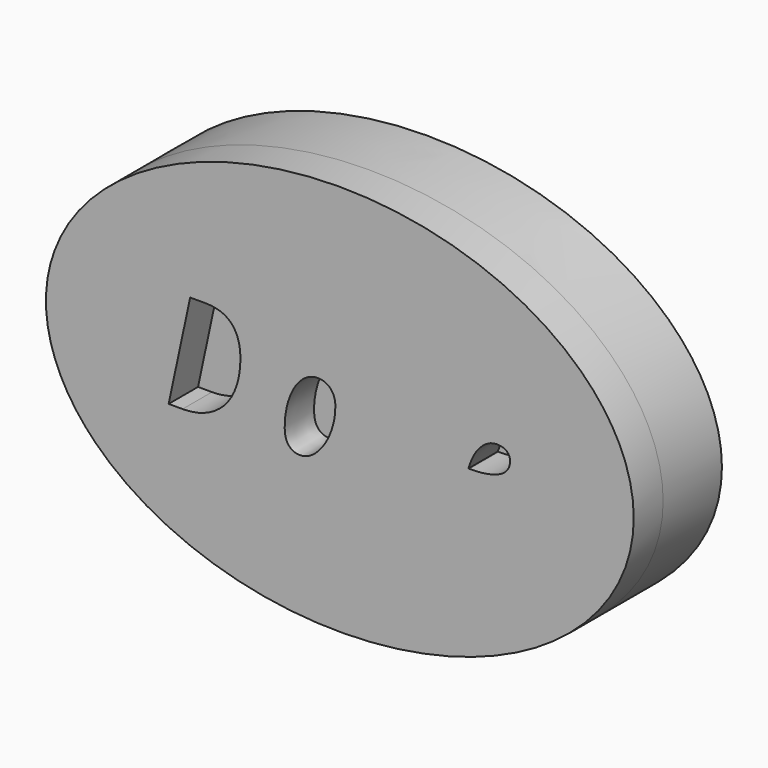
from build123d import *

# Parameters (mm, degrees)
F1_DEPTH     = 9.525
F2_TEXT_SIZE = 22.8748328995
F3_DEPTH     = 4.7625


# Not quite as in the source:
# - Text() gives the source's letters only with a copy of the font that has no kerning and outlines rounded to 1/6400 em; it was checked with that copy


with BuildPart() as f1:
    # F0 (on Front) → F1 (new body)
    with BuildSketch(Plane.XZ):
        with BuildLine():
            add(Edge.make_bspline(
                [(38.1, 0), (38.1, 43.9940905122), (-19.05, 21.9970452561), (-76.2, 0), (-19.05, -21.9970452561), (38.1, -43.9940905122), (38.1, 0)],
                knots=[0, 0, 0, 2.0943951024, 2.0943951024, 4.1887902048, 4.1887902048, 6.2831853072, 6.2831853072, 6.2831853072], degree=2, weights=[1, 0.5, 1, 0.5, 1, 0.5, 1]))
        make_face()
    extrude(amount=-F1_DEPTH)

    # F2 (on face) → F3 (join)
    with BuildSketch(Plane.XZ):
        with BuildLine():
            add(Edge.make_bspline(
                [(38.1, 0), (38.1, 43.9940905122), (-19.05, 21.9970452561), (-76.2, 0), (-19.05, -21.9970452561), (38.1, -43.9940905122), (38.1, 0)],
                knots=[0, 0, 0, 2.0943951024, 2.0943951024, 4.1887902048, 4.1887902048, 6.2831853072, 6.2831853072, 6.2831853072], degree=2, weights=[1, 0.5, 1, 0.5, 1, 0.5, 1]))
        make_face()
        with BuildLine():
            add(Edge.make_bspline(
                [(-12.4810807008, 6.4246112714), (-10.8780553015, 4.7536762119), (-10.8780553015, 1.5619221839)],
                knots=[0, 0, 0, 1, 1, 1], degree=2))
            add(Edge.make_bspline(
                [(-10.8780553015, 1.5619221839), (-10.8780553015, -1.3546190108), (-12.0521775839, -3.5884894111)],
                knots=[0, 0, 0, 1, 1, 1], degree=2))
            add(Edge.make_bspline(
                [(-12.0521775839, -3.5884894111), (-13.2262998663, -5.8223598114), (-15.4029831844, -7.0286498276)],
                knots=[0, 0, 0, 1, 1, 1], degree=2))
            add(Edge.make_bspline(
                [(-15.4029831844, -7.0286498276), (-17.5796665025, -8.2349398438), (-20.5069302751, -8.2349398438)],
                knots=[0, 0, 0, 1, 1, 1], degree=2))
            Line((-20.5069302751, -8.2349398438), (-24.4385421797, -8.2349398438))
            Line((-24.4385421797, -8.2349398438), (-20.9894462816, 8.0955463308))
            Line((-20.9894462816, 8.0955463308), (-17.1686343488, 8.0955463308))
            add(Edge.make_bspline(
                [(-17.1686343488, 8.0955463308), (-14.0841061, 8.0955463308), (-12.4810807008, 6.4246112714)],
                knots=[0, 0, 0, 1, 1, 1], degree=2))
        make_face(mode=Mode.SUBTRACT)
        with BuildLine():
            add(Edge.make_bspline(
                [(-6.0868500668, 3.102399212), (-4.6911278407, 4.2318440864), (-3.0255540702, 4.2318440864)],
                knots=[0, 0, 0, 1, 1, 1], degree=2))
            add(Edge.make_bspline(
                [(-3.0255540702, 4.2318440864), (-1.9997607824, 4.2318440864), (-1.1955674383, 3.6778442271)],
                knots=[0, 0, 0, 1, 1, 1], degree=2))
            add(Edge.make_bspline(
                [(-1.1955674383, 3.6778442271), (-0.3913740941, 3.1238443678), (0.0553999859, 2.0873285021)],
                knots=[0, 0, 0, 1, 1, 1], degree=2))
            Line((0.0553999859, 2.0873285021), (0.1804967283, 2.0873285021))
            Line((0.1804967283, 2.0873285021), (0.9275029902, 4.00666995))
            Line((0.9275029902, 4.00666995), (2.3464574685, 4.00666995))
            Line((2.3464574685, 4.00666995), (-0.2555547738, -8.2349398438))
            Line((-0.2555547738, -8.2349398438), (-1.7424189123, -8.2349398438))
            Line((-1.7424189123, -8.2349398438), (-1.4493351157, -5.9009920495))
            Line((-1.4493351157, -5.9009920495), (-1.5386899318, -5.9009920495))
            add(Edge.make_bspline(
                [(-1.5386899318, -5.9009920495), (-3.5402378105, -8.4601139802), (-5.7526630549, -8.4601139802)],
                knots=[0, 0, 0, 1, 1, 1], degree=2))
            add(Edge.make_bspline(
                [(-5.7526630549, -8.4601139802), (-7.3038626609, -8.4601139802), (-8.1866882432, -7.3539013579)],
                knots=[0, 0, 0, 1, 1, 1], degree=2))
            add(Edge.make_bspline(
                [(-8.1866882432, -7.3539013579), (-9.0695138254, -6.2476887357), (-9.0695138254, -4.3247730951)],
                knots=[0, 0, 0, 1, 1, 1], degree=2))
            add(Edge.make_bspline(
                [(-9.0695138254, -4.3247730951), (-9.0695138254, -2.0015478787), (-8.2760430592, -0.0142967706)],
                knots=[0, 0, 0, 1, 1, 1], degree=2))
            add(Edge.make_bspline(
                [(-8.2760430592, -0.0142967706), (-7.482572293, 1.9729543376), (-6.0868500668, 3.102399212)],
                knots=[0, 0, 0, 1, 1, 1], degree=2))
        make_face(mode=Mode.SUBTRACT)
        with BuildLine():
            Line((7.7971012453, -8.2349398438), (5.2522760853, -8.2349398438))
            Line((5.2522760853, -8.2349398438), (3.8547667628, 4.00666995))
            Line((3.8547667628, 4.00666995), (5.7312178991, 4.00666995))
            Line((5.7312178991, 4.00666995), (6.4460564272, -2.8414831492))
            add(Edge.make_bspline(
                [(6.4460564272, -2.8414831492), (6.7141208753, -5.7222824175), (6.7141208753, -6.8838950257)],
                knots=[0, 0, 0, 1, 1, 1], degree=2))
            Line((6.7141208753, -6.8838950257), (6.7820305354, -6.8838950257))
            add(Edge.make_bspline(
                [(6.7820305354, -6.8838950257), (8.2009850137, -3.8100893548), (8.7800042215, -2.7378315627)],
                knots=[0, 0, 0, 1, 1, 1], degree=2))
            Line((8.7800042215, -2.7378315627), (12.4113839443, 4.00666995))
            Line((12.4113839443, 4.00666995), (14.3986350524, 4.00666995))
            Line((14.3986350524, 4.00666995), (7.7971012453, -8.2349398438))
        make_face(mode=Mode.SUBTRACT)
        with BuildLine():
            add(Edge.make_bspline(
                [(20.5962850911, -8.2635333849), (19.792091747, -8.4601139802), (18.8234855414, -8.4601139802)],
                knots=[0, 0, 0, 1, 1, 1], degree=2))
            add(Edge.make_bspline(
                [(18.8234855414, -8.4601139802), (16.7683247731, -8.4601139802), (15.5942024907, -7.2413142897)],
                knots=[0, 0, 0, 1, 1, 1], degree=2))
            add(Edge.make_bspline(
                [(15.5942024907, -7.2413142897), (14.4200802083, -6.0225145993), (14.4200802083, -3.8672764371)],
                knots=[0, 0, 0, 1, 1, 1], degree=2))
            add(Edge.make_bspline(
                [(14.4200802083, -3.8672764371), (14.4200802083, -1.7692253571), (15.2528670935, 0.1590515725)],
                knots=[0, 0, 0, 1, 1, 1], degree=2))
            add(Edge.make_bspline(
                [(15.2528670935, 0.1590515725), (16.0856539788, 2.0873285021), (17.459931049, 3.1595862942)],
                knots=[0, 0, 0, 1, 1, 1], degree=2))
            add(Edge.make_bspline(
                [(17.459931049, 3.1595862942), (18.8342081193, 4.2318440864), (20.4854851193, 4.2318440864)],
                knots=[0, 0, 0, 1, 1, 1], degree=2))
            add(Edge.make_bspline(
                [(20.4854851193, 4.2318440864), (22.1939492014, 4.2318440864), (23.0553296278, 3.4884120172)],
                knots=[0, 0, 0, 1, 1, 1], degree=2))
            add(Edge.make_bspline(
                [(23.0553296278, 3.4884120172), (23.9167100542, 2.7449799479), (23.9167100542, 1.4153802857)],
                knots=[0, 0, 0, 1, 1, 1], degree=2))
            add(Edge.make_bspline(
                [(23.9167100542, 1.4153802857), (23.9167100542, -0.5933159783), (22.0617040737, -1.7388447196)],
                knots=[0, 0, 0, 1, 1, 1], degree=2))
            add(Edge.make_bspline(
                [(22.0617040737, -1.7388447196), (20.2066980933, -2.8843734609), (16.7540280025, -2.8843734609)],
                knots=[0, 0, 0, 1, 1, 1], degree=2))
            Line((16.7540280025, -2.8843734609), (16.3858861606, -2.8843734609))
            Line((16.3858861606, -2.8843734609), (16.3429958489, -3.7779216211))
            add(Edge.make_bspline(
                [(16.3429958489, -3.7779216211), (16.3429958489, -5.239766411), (17.0292408359, -6.0618307184)],
                knots=[0, 0, 0, 1, 1, 1], degree=2))
            add(Edge.make_bspline(
                [(17.0292408359, -6.0618307184), (17.7154858228, -6.8838950257), (19.155885457, -6.8838950257)],
                knots=[0, 0, 0, 1, 1, 1], degree=2))
            add(Edge.make_bspline(
                [(19.155885457, -6.8838950257), (19.8600014072, -6.8838950257), (20.6034334764, -6.6819531415)],
                knots=[0, 0, 0, 1, 1, 1], degree=2))
            add(Edge.make_bspline(
                [(20.6034334764, -6.6819531415), (21.3468655456, -6.4800112573), (22.4512910716, -5.9438823612)],
                knots=[0, 0, 0, 1, 1, 1], degree=2))
            Line((22.4512910716, -5.9438823612), (22.4512910716, -7.5772883979))
            add(Edge.make_bspline(
                [(22.4512910716, -7.5772883979), (21.4004784352, -8.0669527897), (20.5962850911, -8.2635333849)],
                knots=[0, 0, 0, 1, 1, 1], degree=2))
        make_face(mode=Mode.SUBTRACT)
        with Locations((-25.4, -8.2349398438)):
            Text('Dave', F2_TEXT_SIZE, font='Open Sans', font_style=FontStyle.ITALIC, text_align=(TextAlign.LEFT, TextAlign.BOTTOM))
    extrude(amount=F3_DEPTH)


solid = f1.part
